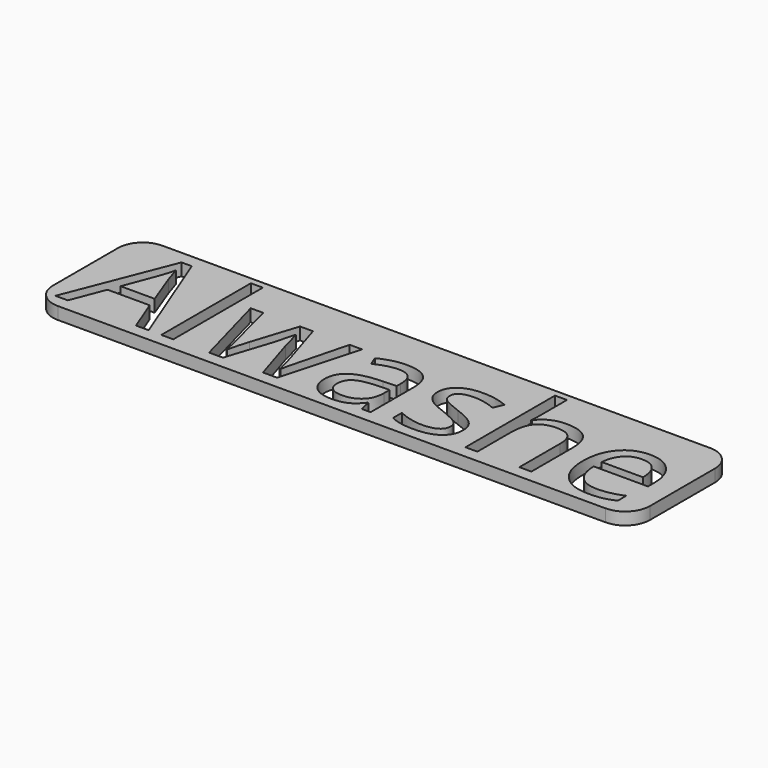
from build123d import *

# Parameters (mm, degrees)
F2_DEPTH     = 1
F0_TEXT_SIZE = 11.9598528795
F3_DEPTH     = 1.001


# Not quite as in the source:
# - Text() gives the source's letters only with a copy of the font that has no kerning and outlines rounded to 1/6400 em; it was checked with that copy


with BuildPart() as f2:
    # F1 (on Top) → F2 (new body)
    with BuildSketch(Plane.XY):
        with BuildLine():
            Line((-22.2264080374, -5.3055470366), (22.2264080374, -5.3055470366))
            ThreePointArc((22.2264080374, -5.3055470366), (23.6406215997, -4.719760599), (24.2264080374, -3.3055470366))
            Line((24.2264080374, -3.3055470366), (24.2264080374, 3.3055470366))
            ThreePointArc((24.2264080374, 3.3055470366), (23.6406215997, 4.719760599), (22.2264080374, 5.3055470366))
            Line((22.2264080374, 5.3055470366), (-22.2264080374, 5.3055470366))
            ThreePointArc((-22.2264080374, 5.3055470366), (-23.6406215997, 4.719760599), (-24.2264080374, 3.3055470366))
            Line((-24.2264080374, 3.3055470366), (-24.2264080374, -3.3055470366))
            ThreePointArc((-24.2264080374, -3.3055470366), (-23.6406215997, -4.719760599), (-22.2264080374, -5.3055470366))
        make_face()
    extrude(amount=-F2_DEPTH)

    # F0 (on Top) → F3 (cut, through all)
    with BuildSketch(Plane.XY):
        with Locations((-23.2264080374, -4.3055470366)):
            Text('Alwashe', F0_TEXT_SIZE, font='Open Sans', text_align=(TextAlign.LEFT, TextAlign.BOTTOM))
    extrude(amount=-F3_DEPTH, mode=Mode.SUBTRACT)


solid = f2.part
